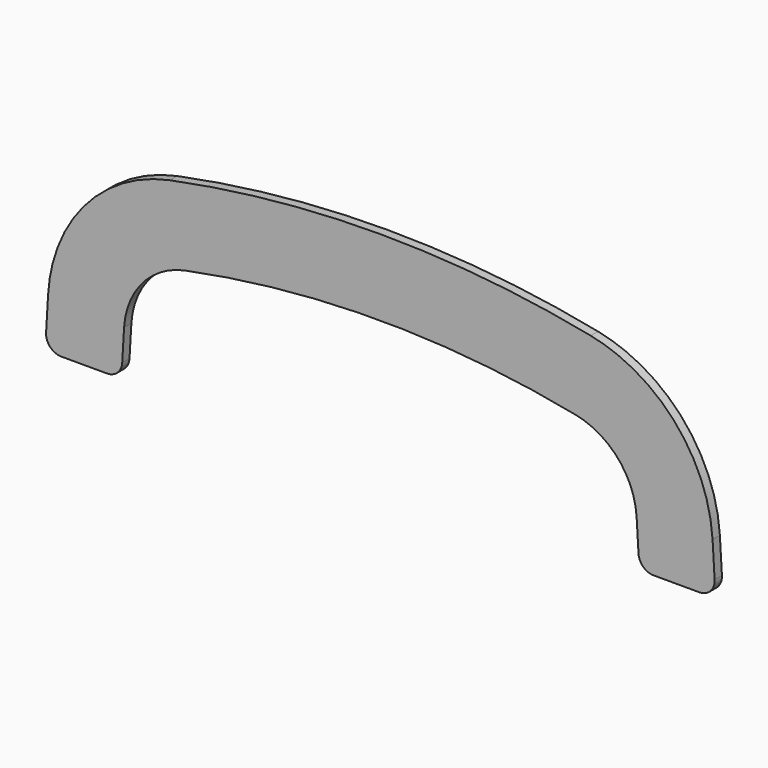
from build123d import *

# Parameters (mm, degrees)
F1_DEPTH = 18
F2_R     = 300
F4_DEPTH = 18.0010001
F5_R     = 30


# Not quite as in the source:
# - a feature names something its author has since deleted; it is built from what else it names


with BuildPart() as f1:
    # F0 (on Front) → F1 (new body)
    with BuildSketch(Plane.XZ):
        with BuildLine():
            Line((-685, 200), (-685, 0))
            Line((-685, 0), (685, 0))
            Line((685, 0), (685, 200))
            ThreePointArc((685, 200), (673.7460477003, 800.4217267888), (640, 1400))
            ThreePointArc((640, 1400), (0, 1500), (-640, 1400))
            ThreePointArc((-640, 1400), (-673.7460477003, 800.4217267888), (-685, 200))
        make_face()
    extrude(amount=F1_DEPTH)

    # F2
    f2_edges = [f1.edges().sort_by_distance(p)[0] for p in [
        (-640, -9, 1400),
        (640, -9, 1400),
    ]]
    fillet(f2_edges, radius=F2_R)

    # F3 (on face) → F4 (cut, through all)
    with BuildSketch(Plane.XZ.offset(18)):
        with BuildLine():
            ThreePointArc((-385.0351790184, 1311.5685143294), (-468.492433607, 1263.0523750474), (-505.1041546871, 1173.7298639214))
            ThreePointArc((-505.1041546871, 1173.7298639214), (-507.8289943623, 1128.3346974136), (-510.4237596585, 1082.9319102019))
            Line((-510.4237596585, 1082.9319102019), (-660.6541901542, 1082.9319102019))
            ThreePointArc((-660.6541901542, 1082.9319102019), (-678.9123910716, 641.6337499869), (-685, 200))
            Line((-685, 200), (-685, 0))
            Line((-685, 0), (685, 0))
            Line((685, 0), (685, 200))
            ThreePointArc((685, 200), (678.9123910716, 641.6337499869), (660.6541901542, 1082.9319102019))
            Line((660.6541901542, 1082.9319102019), (510.4237596585, 1082.9319102019))
            ThreePointArc((510.4237596585, 1082.9319102019), (507.8289943623, 1128.3346974136), (505.1041546871, 1173.7298639214))
            ThreePointArc((505.1041546871, 1173.7298639214), (468.492433607, 1263.0523750474), (385.0351790184, 1311.5685143294))
            ThreePointArc((385.0351790184, 1311.5685143294), (0, 1350), (-385.0351790184, 1311.5685143294))
        make_face()
    extrude(amount=-F4_DEPTH, mode=Mode.SUBTRACT)

    # F5
    f5_edges = [f1.edges().sort_by_distance(p)[0] for p in [
        (-510.42376, -9, 1082.93191),
        (510.42376, -9, 1082.93191),
        (-660.65419, -9, 1082.93191),
        (660.65419, -9, 1082.93191),
    ]]
    fillet(f5_edges, radius=F5_R)


solid = f1.part
